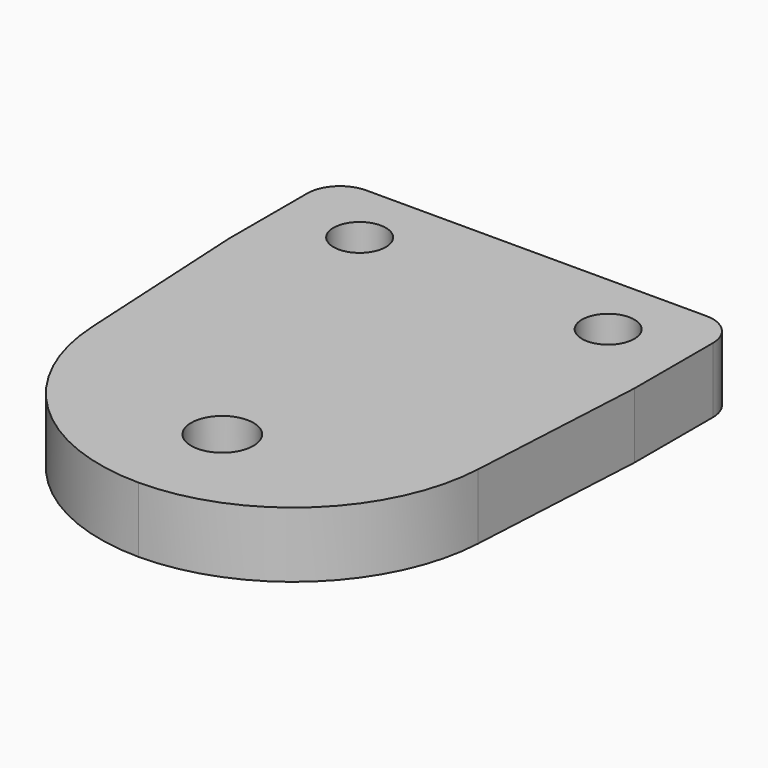
from build123d import *

# Parameters (mm, degrees)
F0_W        = 56
F0_H        = 76
F1_DEPTH    = 10
F2_D        = 9.525
F3_T1_DEPTH = 150.1699053678
F4_R        = 5
F5_D        = 8


# Not quite as in the source:
# - a fillet or chamfer that OpenCascade refuses, or shapes differently, is made with other operations: its cross-section is extruded or revolved along the edge and cut away or added
# - a length typed as a fraction of an inch, garbled in the dataset ("3 / 203.2 mm" for 3/8 in), is restored


with BuildPart() as f1:
    # F0 (on Top) → F1 (new body)
    with BuildSketch(Plane.XY):
        Rectangle(F0_W, F0_H)
        Polygon((-31, 18), (-28, -38), (-28, 38), (-31, 38), align=None)
        Polygon((28, 38), (28, -38), (31, 18), (31, 38), align=None)
    extrude(amount=-F1_DEPTH)

    # F2 (through all)
    with Locations(Plane.XY):
        with Locations((0, -22)):
            Hole(F2_D / 2)

    # F3: fillet of radius 29.576 on 2 edges, made by hand

    # F3_s2 → F3_t1 (cut)
    with BuildSketch(Plane.XY.offset(-80.0849526839)):
        with BuildLine():
            ThreePointArc((-0.0339810736, -38), (20.3123431081, -29.889480854), (29.4996700065, -10.0061598793))
            Line((29.4996700065, -10.0061598793), (28, -38))
            Line((28, -38), (-0.0339810736, -38))
        make_face()
        with BuildLine():
            ThreePointArc((0.0339810736, -38), (-20.3123431081, -29.889480854), (-29.4996700065, -10.0061598793))
            Line((-29.4996700065, -10.0061598793), (-28, -38))
            Line((-28, -38), (0.0339810736, -38))
        make_face()
    extrude(amount=F3_T1_DEPTH, mode=Mode.SUBTRACT)

    # F4
    f4_edges = [f1.edges().sort_by_distance(p)[0] for p in [
        (-31, 38, -5),
        (31, 38, -5),
    ]]
    fillet(f4_edges, radius=F4_R)

    # F5 (through all)
    with Locations(Plane.XY):
        with Locations((-19, 28), (19, 28)):
            Hole(F5_D / 2)


solid = f1.part
